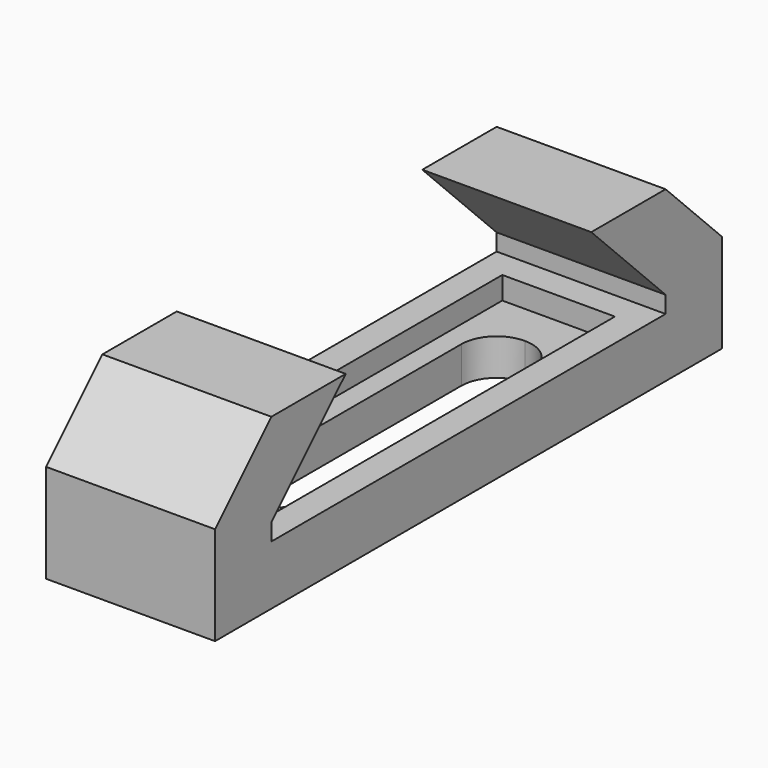
from build123d import *

# Parameters (mm, degrees)
F0_W     = 12
F0_H     = 45
F1_DEPTH = 12
F2_W     = 35
F2_H     = 1.2
F3_DEPTH = 12
F4_SIZE  = 5
F5_W     = 8
F5_H     = 31
F6_DEPTH = 1.6
F7_W     = 5
F7_H     = 25
F8_DEPTH = 2.6
F9_R     = 2.49999


# Not quite as in the source:
# - a fillet or chamfer is up to 0.001 mm smaller than in the source, because OpenCascade refuses the exact size


with BuildPart() as f1:
    # F0 (on Top) → F1 (new body)
    with BuildSketch(Plane.XY):
        Rectangle(F0_W, F0_H)
    extrude(amount=F1_DEPTH)

    # F2 (on face) → F3 (cut, through all)
    with BuildSketch(Plane(origin=(-6, 0, 0), x_dir=(0, -1, 0), z_dir=(-1, 0, 0))):
        Polygon((-17.5, 5.4), (17.5, 5.4), (10.9, 12), (-10.9, 12), align=None)
        with Locations((0, 4.8)):
            Rectangle(F2_W, F2_H)
    extrude(amount=-F3_DEPTH, mode=Mode.SUBTRACT)

    # F4
    f4_edges = [f1.edges().sort_by_distance(p)[0] for p in [
        (0, 22.5, 12),
        (0, -22.5, 12),
    ]]
    chamfer(f4_edges, length=F4_SIZE)

    # F5 (on face) → F6 (cut)
    with BuildSketch(Plane.XY.offset(4.2)):
        Rectangle(F5_W, F5_H)
    extrude(amount=-F6_DEPTH, mode=Mode.SUBTRACT)

    # F7 (on face) → F8 (cut, through all)
    with BuildSketch(Plane.XY.offset(2.6)):
        Rectangle(F7_W, F7_H)
    extrude(amount=-F8_DEPTH, mode=Mode.SUBTRACT)

    # F9 (radius 2.5 in the source; OpenCascade refuses exactly that, so slightly less here)
    f9_edges = [f1.edges().sort_by_distance(p)[0] for p in [
        (2.5, 12.5, 1.3),
        (-2.5, 12.5, 1.3),
        (-2.5, -12.5, 1.3),
        (2.5, -12.5, 1.3),
    ]]
    fillet(f9_edges, radius=F9_R)


solid = f1.part
